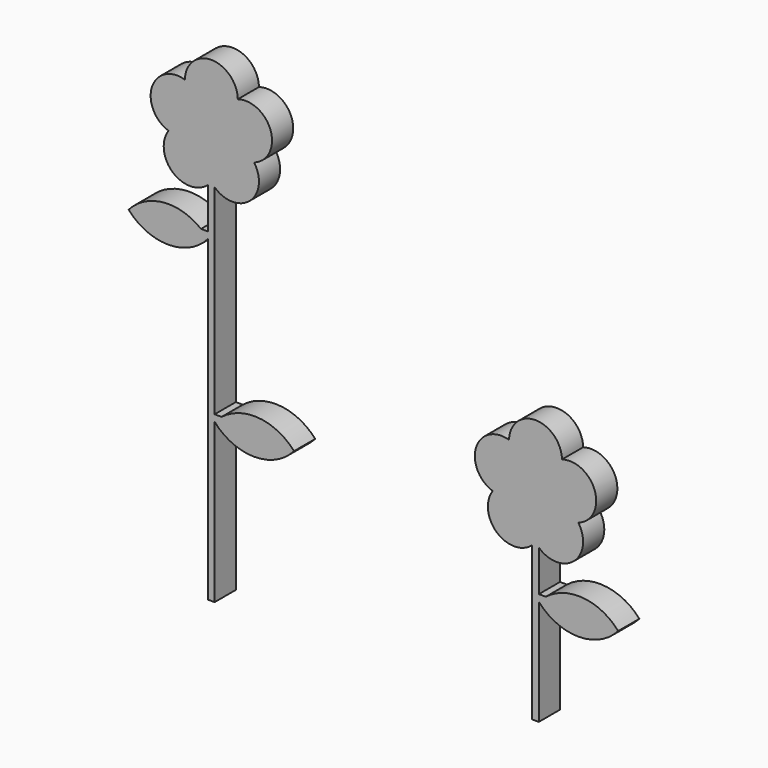
from build123d import *

# Parameters (mm, degrees)
F1_DEPTH = 25.4


with BuildPart() as f1:
    # F0 (on Front) → F1 (new body)
    with BuildSketch(Plane.XZ):
        with BuildLine():
            ThreePointArc((-44.2678929043, 383.8952975035), (-40.260109895, 350.2213176653), (-6.35, 350.5433265189))
            Line((-6.35, 350.5433265189), (-6.35, 359.6170129621))
            ThreePointArc((-6.35, 359.6170129621), (-8.2653665538, 369.2933754965), (-6.35, 378.9697380309))
            ThreePointArc((-6.35, 378.9697380309), (-4.9393657292, 381.8591448881), (-3.175, 384.5471877833))
            ThreePointArc((-3.175, 384.5471877833), (-1.4106342708, 381.8591448881), (0, 378.9697380309))
            ThreePointArc((0, 378.9697380309), (1.9153665538, 369.2933754965), (0, 359.6170129621))
            Line((0, 359.6170129621), (0, 350.5433265189))
            ThreePointArc((0, 350.5433265189), (33.910109895, 350.2213176653), (37.9178929043, 383.8952975035))
            ThreePointArc((37.9178929043, 383.8952975035), (53.8435127289, 415.7736256188), (22.2218045109, 432.2028903499))
            ThreePointArc((22.2218045109, 432.2028903499), (-3.175, 457.2), (-28.5718045109, 432.2028903499))
            ThreePointArc((-28.5718045109, 432.2028903499), (-60.1935127289, 415.7736256188), (-44.2678929043, 383.8952975035))
        make_face()
        with BuildLine():
            ThreePointArc((-15.2534177569, 393.3226719547), (-28.1876455579, 383.7677584478), (-44.2678929043, 383.8952975035))
            ThreePointArc((-44.2678929043, 383.8952975035), (-31.3336651033, 393.4502110104), (-15.2534177569, 393.3226719547))
        make_face(mode=Mode.SUBTRACT)
        with BuildLine():
            ThreePointArc((8.9034177569, 393.3226719547), (24.9836651033, 393.4502110104), (37.9178929043, 383.8952975035))
            ThreePointArc((37.9178929043, 383.8952975035), (21.8376455579, 383.7677584478), (8.9034177569, 393.3226719547))
        make_face(mode=Mode.SUBTRACT)
        with BuildLine():
            ThreePointArc((-10.6398727041, 407.5217036118), (-23.7240316571, 416.8702545918), (-28.5718045109, 432.2028903499))
            ThreePointArc((-28.5718045109, 432.2028903499), (-15.4876455579, 422.8543393699), (-10.6398727041, 407.5217036118))
        make_face(mode=Mode.SUBTRACT)
        with BuildLine():
            ThreePointArc((4.2898727041, 407.5217036118), (9.1376455579, 422.8543393699), (22.2218045109, 432.2028903499))
            ThreePointArc((22.2218045109, 432.2028903499), (17.3740316571, 416.8702545918), (4.2898727041, 407.5217036118))
        make_face(mode=Mode.SUBTRACT)
        with BuildLine():
            Line((-6.35, 304.8), (-6.35, 0))
            Line((-6.35, 0), (0, 0))
            Line((0, 0), (0, 152.4))
            Line((0, 152.4), (0, 158.75))
            Line((0, 158.75), (0, 350.5433265189))
            ThreePointArc((0, 350.5433265189), (-1.6689353248, 352.2174918745), (-3.175, 354.0395632097))
            ThreePointArc((-3.175, 354.0395632097), (-4.6810646752, 352.2174918745), (-6.35, 350.5433265189))
            Line((-6.35, 350.5433265189), (-6.35, 311.15))
            Line((-6.35, 311.15), (-6.35, 304.8))
        make_face()
        with BuildLine():
            ThreePointArc((-82.55, 304.8), (-44.45, 287.6010416505), (-6.35, 304.8))
            ThreePointArc((-6.35, 304.8), (-9.56640613, 308.1282810987), (-13.0723922034, 311.15))
            ThreePointArc((-13.0723922034, 311.15), (-49.0736635079, 321.7881047721), (-82.55, 304.8))
        make_face()
        with BuildLine():
            ThreePointArc((6.7223922034, 158.75), (3.21640613, 155.7282810987), (0, 152.4))
            ThreePointArc((0, 152.4), (38.1, 135.2010416505), (76.2, 152.4))
            ThreePointArc((76.2, 152.4), (42.7236635079, 169.3881047721), (6.7223922034, 158.75))
        make_face()
        with BuildLine():
            ThreePointArc((8.9034177569, 393.3226719547), (21.8376455579, 383.7677584478), (37.9178929043, 383.8952975035))
            ThreePointArc((37.9178929043, 383.8952975035), (24.9836651033, 393.4502110104), (8.9034177569, 393.3226719547))
        make_face()
        with BuildLine():
            ThreePointArc((4.2898727041, 407.5217036118), (17.3740316571, 416.8702545918), (22.2218045109, 432.2028903499))
            ThreePointArc((22.2218045109, 432.2028903499), (9.1376455579, 422.8543393699), (4.2898727041, 407.5217036118))
        make_face()
        with BuildLine():
            ThreePointArc((-10.6398727041, 407.5217036118), (-15.4876455579, 422.8543393699), (-28.5718045109, 432.2028903499))
            ThreePointArc((-28.5718045109, 432.2028903499), (-23.7240316571, 416.8702545918), (-10.6398727041, 407.5217036118))
        make_face()
        with BuildLine():
            ThreePointArc((-15.2534177569, 393.3226719547), (-31.3336651033, 393.4502110104), (-44.2678929043, 383.8952975035))
            ThreePointArc((-44.2678929043, 383.8952975035), (-28.1876455579, 383.7677584478), (-15.2534177569, 393.3226719547))
        make_face()
        with BuildLine():
            Line((-6.35, 378.9697380309), (-6.35, 359.6170129621))
            ThreePointArc((-6.35, 359.6170129621), (-4.9393657292, 356.7276061049), (-3.175, 354.0395632097))
            ThreePointArc((-3.175, 354.0395632097), (-1.4106342708, 356.7276061049), (0, 359.6170129621))
            Line((0, 359.6170129621), (0, 378.9697380309))
            ThreePointArc((0, 378.9697380309), (-1.4106342708, 381.8591448881), (-3.175, 384.5471877833))
            ThreePointArc((-3.175, 384.5471877833), (-4.9393657292, 381.8591448881), (-6.35, 378.9697380309))
        make_face()
        with BuildLine():
            ThreePointArc((-6.35, 378.9697380309), (-8.2653665538, 369.2933754965), (-6.35, 359.6170129621))
            Line((-6.35, 359.6170129621), (-6.35, 378.9697380309))
        make_face()
        with BuildLine():
            Line((0, 378.9697380309), (0, 359.6170129621))
            ThreePointArc((0, 359.6170129621), (1.9153665538, 369.2933754965), (0, 378.9697380309))
        make_face()
        with BuildLine():
            ThreePointArc((-13.0723922034, 311.15), (-9.56640613, 308.1282810987), (-6.35, 304.8))
            Line((-6.35, 304.8), (-6.35, 311.15))
            Line((-6.35, 311.15), (-13.0723922034, 311.15))
        make_face()
        with BuildLine():
            Line((0, 158.75), (0, 152.4))
            ThreePointArc((0, 152.4), (3.21640613, 155.7282810987), (6.7223922034, 158.75))
            Line((6.7223922034, 158.75), (0, 158.75))
        make_face()
        with BuildLine():
            Line((-6.35, 359.6170129621), (-6.35, 350.5433265189))
            ThreePointArc((-6.35, 350.5433265189), (-4.6810646752, 352.2174918745), (-3.175, 354.0395632097))
            ThreePointArc((-3.175, 354.0395632097), (-4.9393657292, 356.7276061049), (-6.35, 359.6170129621))
        make_face()
        with BuildLine():
            ThreePointArc((0, 359.6170129621), (-1.4106342708, 356.7276061049), (-3.175, 354.0395632097))
            ThreePointArc((-3.175, 354.0395632097), (-1.6689353248, 352.2174918745), (0, 350.5433265189))
            Line((0, 350.5433265189), (0, 359.6170129621))
        make_face()
    extrude(amount=F1_DEPTH)


with BuildPart() as f1b:
    # F0 (on Front) → F1, piece 2 (new body)
    with BuildSketch(Plane.XZ):
        with BuildLine():
            ThreePointArc((266.8821070957, 180.6952975035), (270.889890105, 147.0213176653), (304.8, 147.3433265189))
            Line((304.8, 147.3433265189), (304.8, 156.4170129621))
            ThreePointArc((304.8, 156.4170129621), (302.8846334462, 166.0933754965), (304.8, 175.7697380309))
            ThreePointArc((304.8, 175.7697380309), (306.2106342708, 178.6591448881), (307.975, 181.3471877833))
            ThreePointArc((307.975, 181.3471877833), (309.7393657292, 178.6591448881), (311.15, 175.7697380309))
            ThreePointArc((311.15, 175.7697380309), (313.0653665538, 166.0933754965), (311.15, 156.4170129621))
            Line((311.15, 156.4170129621), (311.15, 147.3433265189))
            ThreePointArc((311.15, 147.3433265189), (345.060109895, 147.0213176653), (349.0678929043, 180.6952975035))
            ThreePointArc((349.0678929043, 180.6952975035), (364.9935127289, 212.5736256188), (333.3718045109, 229.0028903499))
            ThreePointArc((333.3718045109, 229.0028903499), (307.975, 254), (282.5781954891, 229.0028903499))
            ThreePointArc((282.5781954891, 229.0028903499), (250.9564872711, 212.5736256188), (266.8821070957, 180.6952975035))
        make_face()
        with BuildLine():
            ThreePointArc((295.8965822431, 190.1226719547), (282.9623544421, 180.5677584478), (266.8821070957, 180.6952975035))
            ThreePointArc((266.8821070957, 180.6952975035), (279.8163348967, 190.2502110104), (295.8965822431, 190.1226719547))
        make_face(mode=Mode.SUBTRACT)
        with BuildLine():
            ThreePointArc((300.5101272959, 204.3217036118), (287.4259683429, 213.6702545918), (282.5781954891, 229.0028903499))
            ThreePointArc((282.5781954891, 229.0028903499), (295.6623544421, 219.6543393699), (300.5101272959, 204.3217036118))
        make_face(mode=Mode.SUBTRACT)
        with BuildLine():
            ThreePointArc((315.4398727041, 204.3217036118), (320.2876455579, 219.6543393699), (333.3718045109, 229.0028903499))
            ThreePointArc((333.3718045109, 229.0028903499), (328.5240316571, 213.6702545918), (315.4398727041, 204.3217036118))
        make_face(mode=Mode.SUBTRACT)
        with BuildLine():
            ThreePointArc((320.0534177569, 190.1226719547), (336.1336651033, 190.2502110104), (349.0678929043, 180.6952975035))
            ThreePointArc((349.0678929043, 180.6952975035), (332.9876455579, 180.5677584478), (320.0534177569, 190.1226719547))
        make_face(mode=Mode.SUBTRACT)
        with BuildLine():
            ThreePointArc((317.8723922034, 107.95), (314.36640613, 104.9282810987), (311.15, 101.6))
            ThreePointArc((311.15, 101.6), (349.25, 84.4010416505), (387.35, 101.6))
            ThreePointArc((387.35, 101.6), (353.8736635079, 118.5881047721), (317.8723922034, 107.95))
        make_face()
        with BuildLine():
            Line((304.8, 147.3433265189), (304.8, 0))
            Line((304.8, 0), (311.15, 0))
            Line((311.15, 0), (311.15, 101.6))
            Line((311.15, 101.6), (311.15, 107.95))
            Line((311.15, 107.95), (311.15, 147.3433265189))
            ThreePointArc((311.15, 147.3433265189), (309.4810646752, 149.0174918745), (307.975, 150.8395632097))
            ThreePointArc((307.975, 150.8395632097), (306.4689353248, 149.0174918745), (304.8, 147.3433265189))
        make_face()
        with BuildLine():
            ThreePointArc((320.0534177569, 190.1226719547), (332.9876455579, 180.5677584478), (349.0678929043, 180.6952975035))
            ThreePointArc((349.0678929043, 180.6952975035), (336.1336651033, 190.2502110104), (320.0534177569, 190.1226719547))
        make_face()
        with BuildLine():
            ThreePointArc((315.4398727041, 204.3217036118), (328.5240316571, 213.6702545918), (333.3718045109, 229.0028903499))
            ThreePointArc((333.3718045109, 229.0028903499), (320.2876455579, 219.6543393699), (315.4398727041, 204.3217036118))
        make_face()
        with BuildLine():
            ThreePointArc((300.5101272959, 204.3217036118), (295.6623544421, 219.6543393699), (282.5781954891, 229.0028903499))
            ThreePointArc((282.5781954891, 229.0028903499), (287.4259683429, 213.6702545918), (300.5101272959, 204.3217036118))
        make_face()
        with BuildLine():
            ThreePointArc((295.8965822431, 190.1226719547), (279.8163348967, 190.2502110104), (266.8821070957, 180.6952975035))
            ThreePointArc((266.8821070957, 180.6952975035), (282.9623544421, 180.5677584478), (295.8965822431, 190.1226719547))
        make_face()
        with BuildLine():
            Line((304.8, 175.7697380309), (304.8, 156.4170129621))
            ThreePointArc((304.8, 156.4170129621), (306.2106342708, 153.5276061049), (307.975, 150.8395632097))
            ThreePointArc((307.975, 150.8395632097), (309.7393657292, 153.5276061049), (311.15, 156.4170129621))
            Line((311.15, 156.4170129621), (311.15, 175.7697380309))
            ThreePointArc((311.15, 175.7697380309), (309.7393657292, 178.6591448881), (307.975, 181.3471877833))
            ThreePointArc((307.975, 181.3471877833), (306.2106342708, 178.6591448881), (304.8, 175.7697380309))
        make_face()
        with BuildLine():
            ThreePointArc((304.8, 175.7697380309), (302.8846334462, 166.0933754965), (304.8, 156.4170129621))
            Line((304.8, 156.4170129621), (304.8, 175.7697380309))
        make_face()
        with BuildLine():
            Line((311.15, 175.7697380309), (311.15, 156.4170129621))
            ThreePointArc((311.15, 156.4170129621), (313.0653665538, 166.0933754965), (311.15, 175.7697380309))
        make_face()
        with BuildLine():
            Line((311.15, 107.95), (311.15, 101.6))
            ThreePointArc((311.15, 101.6), (314.36640613, 104.9282810987), (317.8723922034, 107.95))
            Line((317.8723922034, 107.95), (311.15, 107.95))
        make_face()
        with BuildLine():
            Line((304.8, 156.4170129621), (304.8, 147.3433265189))
            ThreePointArc((304.8, 147.3433265189), (306.4689353248, 149.0174918745), (307.975, 150.8395632097))
            ThreePointArc((307.975, 150.8395632097), (306.2106342708, 153.5276061049), (304.8, 156.4170129621))
        make_face()
        with BuildLine():
            ThreePointArc((311.15, 156.4170129621), (309.7393657292, 153.5276061049), (307.975, 150.8395632097))
            ThreePointArc((307.975, 150.8395632097), (309.4810646752, 149.0174918745), (311.15, 147.3433265189))
            Line((311.15, 147.3433265189), (311.15, 156.4170129621))
        make_face()
    extrude(amount=F1_DEPTH)


solid = Compound([f1.part, f1b.part])
